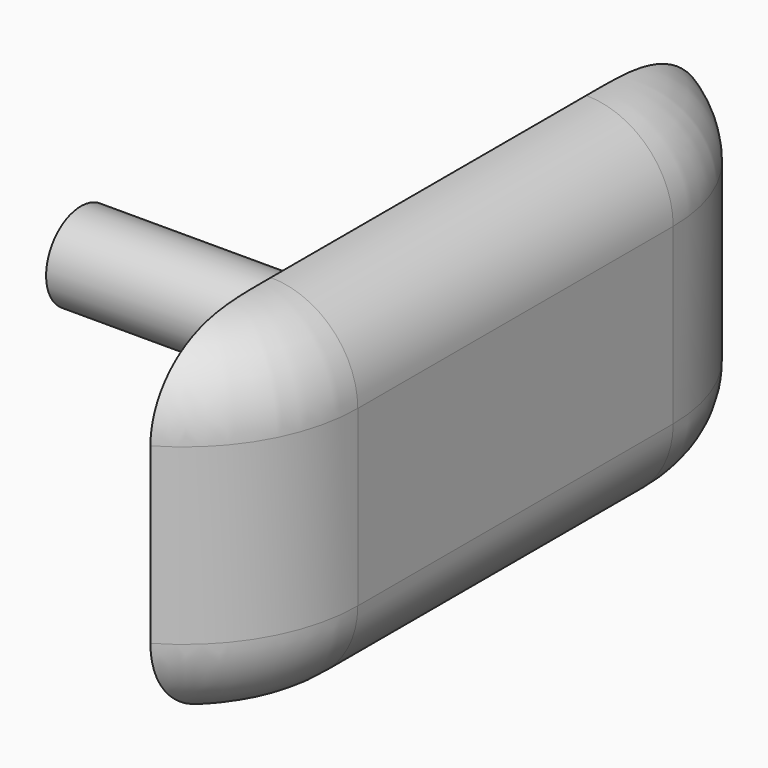
from build123d import *

# Parameters (mm, degrees)
F0_W        = 1.27
F0_H        = 10.16
F1_DEPTH    = 5.08
F2_T1_DEPTH = 16.0785226281
F3_R        = 1.26999
F4_R        = 0.635
F5_DEPTH    = 5.08


# Not quite as in the source:
# - a fillet or chamfer that OpenCascade refuses, or shapes differently, is made with other operations: its cross-section is extruded or revolved along the edge and cut away or added
# - a fillet or chamfer is up to 0.001 mm smaller than in the source, because OpenCascade refuses the exact size


with BuildPart() as f1:
    # F0 (on Top) → F1 (new body)
    with BuildSketch(Plane.XY):
        with Locations((0.635, 2.7667839336)):
            Rectangle(F0_W, F0_H)
    extrude(amount=F1_DEPTH)

    # F2: fillet of radius 2.54 on 2 edges, made by hand

    # F2_s2 → F2_t1 (cut)
    with BuildSketch(Plane.XY.offset(-5.499261314)):
        with BuildLine():
            ThreePointArc((0, 7.8467839336), (0.9297045256, 6.9170794079), (1.27, 5.6470794079))
            Line((1.27, 5.6470794079), (1.27, 7.8467839336))
            Line((1.27, 7.8467839336), (0, 7.8467839336))
        make_face()
        with BuildLine():
            ThreePointArc((0, -2.3132160664), (0.9297045256, -1.3835115408), (1.27, -0.1135115408))
            Line((1.27, -0.1135115408), (1.27, -2.3132160664))
            Line((1.27, -2.3132160664), (0, -2.3132160664))
        make_face()
    extrude(amount=F2_T1_DEPTH, mode=Mode.SUBTRACT)

    # F3 (radius 1.27 in the source; OpenCascade refuses exactly that, so slightly less here)
    f3_edges = [f1.edges().sort_by_distance(p)[0] for p in [
        (0.929705, 6.917079, 5.08),
        (1.27, 2.766784, 5.08),
        (0.929705, -1.383512, 5.08),
        (0.929705, 6.917079, 0),
        (0.929705, -1.383512, 0),
        (1.27, 2.766784, 0),
    ]]
    fillet(f3_edges, radius=F3_R)

    # F4 (on face) → F5 (join)
    with BuildSketch(Plane(origin=(0, 0, 0), x_dir=(0, -1, 0), z_dir=(-1, 0, 0))):
        with Locations((-2.7667839336, 2.54)):
            Circle(F4_R)
    extrude(amount=F5_DEPTH)


solid = f1.part
